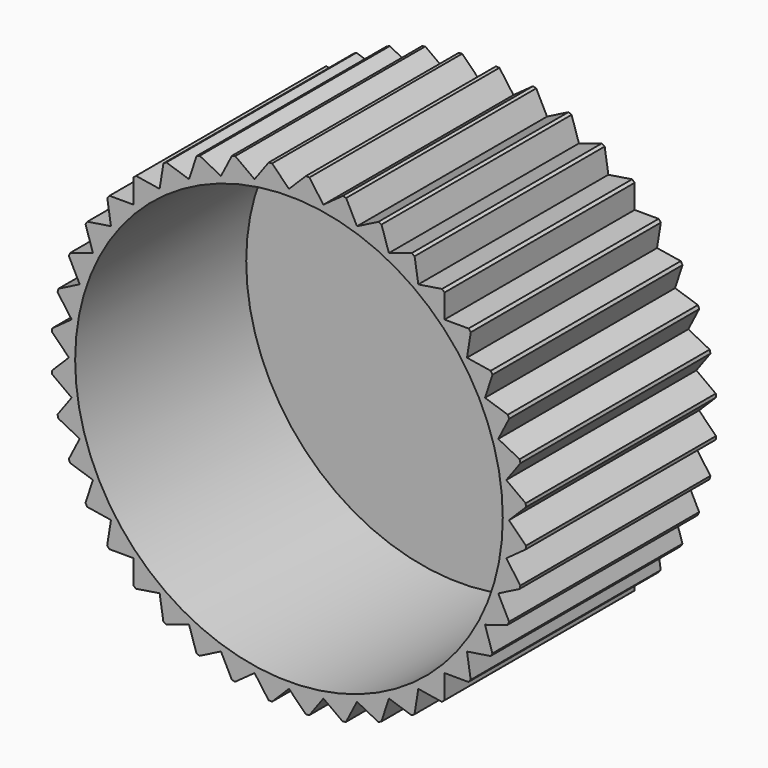
from build123d import *

# Parameters (mm, degrees)
F0_R            = 25.4
F1_DEPTH        = 25.4
F2_T            = -2.54
F6_DEPTH        = 25.4
F6_COPIES_COUNT = 40


# Not quite as in the source:
# - a pattern or mirror of a feature is missing from the dataset's text; its kind, count and spacing are read off the source's solid
# - a feature names something its author has since deleted; it is built from what else it names


with BuildPart() as f1:
    # F0 (on Front) → F1 (new body)
    with BuildSketch(Plane.XZ):
        Circle(F0_R)
    extrude(amount=F1_DEPTH)

    # F2
    f2_openings = [f1.faces().sort_by_distance(p)[0] for p in [
        (0, -25.4, 0),
    ]]
    offset(amount=F2_T, openings=f2_openings)

    # F4 (on offset) → F6 (cut)
    with BuildSketch(Plane.XZ.offset(25.4)):
        Polygon((1.9352714298, 25.4522323095), (-1.9276905805, 25.4598131588), (0, 23.524541729), align=None)
    f6 = extrude(amount=-F6_DEPTH, mode=Mode.SUBTRACT)

    # F6_copies: F6 ×40 about axis
    f6_copies_axis = Axis((0, 0, 0), (0, 1, 0))
    for i in range(1, F6_COPIES_COUNT):
        add(f6.rotate(f6_copies_axis, i * 360 / F6_COPIES_COUNT), mode=Mode.SUBTRACT)


solid = f1.part
